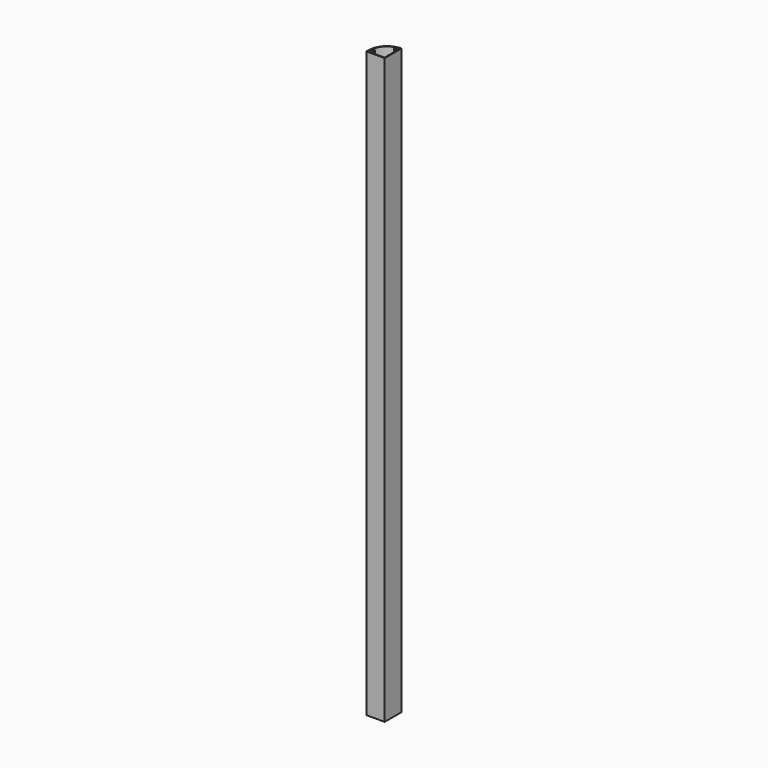
from build123d import *

# Parameters (mm, degrees)
F1_DEPTH = 1320


# Not quite as in the source:
# - ends of sketch curves that miss each other by under 0.0002 mm in the source are joined


with BuildPart() as f1:
    # F0 (on Top) → F1 (new body)
    with BuildSketch(Plane.XY):
        with BuildLine():
            Line((0.0702818, 6.4022224), (0.0702818, 0.0522224))
            Line((0.0702818, 0.0522224), (41.3452818, 0.0522224))
            Line((41.3452818, 0.0522224), (41.3452818, 47.6772224))
            ThreePointArc((41.3452818, 47.6772224), (12.1594494065, 35.5880547935), (0.0702818, 6.4022224))
        make_face()
        with BuildLine():
            ThreePointArc((2.4627294682, 14.0316719322), (12.0103779586, 33.0391289887), (30.0113989636, 44.370689262))
            ThreePointArc((30.0113989636, 44.370689262), (31.5911647015, 43.7909818691), (31.4826885527, 42.111702976))
            ThreePointArc((31.4826885527, 42.111702976), (30.7556005021, 40.0197952956), (31.6365393769, 37.9878855663))
            ThreePointArc((31.6365393769, 37.9878855663), (32.5345549665, 37.9838460356), (32.5385935644, 38.8818625665))
            ThreePointArc((32.5385935644, 38.8818625665), (33.8014907398, 41.9114224), (35.0643565086, 38.8818507998))
            ThreePointArc((35.0643565086, 38.8818507998), (35.0683832335, 37.9838460356), (35.9663997644, 37.9878846335))
            ThreePointArc((35.9663997644, 37.9878846335), (36.7987348031, 40.6872982302), (35.056647343, 42.9109867034))
            ThreePointArc((35.056647343, 42.9109867034), (34.2431436666, 44.3840647436), (35.4254562981, 45.581518551))
            ThreePointArc((35.4254562981, 45.581518551), (37.5543147935, 45.8444579497), (39.6942825983, 45.9918116582))
            Line((39.6942825983, 45.9918116582), (39.6942818, 1.7032224))
            Line((39.6942818, 1.7032224), (1.7212818, 1.7032224))
            Line((1.7212818, 1.7032224), (1.7212818, 6.4022224))
            ThreePointArc((1.7212818, 6.4022224), (1.7261013466, 7.0202160926), (1.7405588141, 7.6380594495))
            ThreePointArc((1.7405588141, 7.6380594495), (3.0583454152, 9.3170447758), (5.0535040361, 8.5588069696))
            ThreePointArc((5.0535040361, 8.5588069696), (7.2847284354, 7.1820688789), (9.7596313332, 8.0472925626))
            ThreePointArc((9.7596313332, 8.0472925626), (9.7636581644, 8.9453209665), (8.8656416335, 8.9493595644))
            ThreePointArc((8.8656416335, 8.9493595644), (5.8360818, 10.2122134602), (8.8656407007, 11.4751096943))
            ThreePointArc((8.8656407007, 11.4751096943), (9.7636581644, 11.4791492335), (9.7596195665, 12.3771657644))
            ThreePointArc((9.7596195665, 12.3771657644), (7.6269060344, 13.2601954214), (5.4868384376, 12.3951423887))
            ThreePointArc((5.4868384376, 12.3951423887), (3.3728152631, 12.1010480384), (2.4627294682, 14.0316719322))
        make_face(mode=Mode.SUBTRACT)
    extrude(amount=F1_DEPTH)


solid = f1.part
